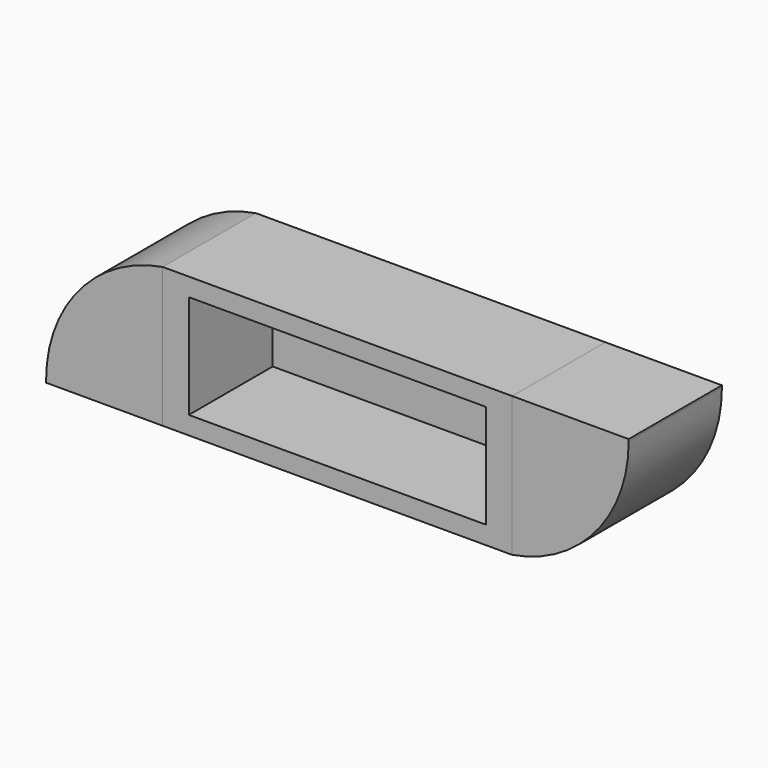
from build123d import *

# Parameters (mm, degrees)
F0_W          = 25.5
F0_H          = 8.9
F1_DEPTH      = 8.9
F2_W          = 30
F2_H          = 12
F2_W_2        = 25.5
F2_H_2        = 8.9
F3_DEPTH      = 10
F4_DEPTH      = 9
F5_DEPTH      = 10
F6_DEPTH      = 10
F9_T1_DEPTH   = 69.160797831
F9_2_T1_DEPTH = 69.160797831


# Not quite as in the source:
# - a fillet or chamfer that OpenCascade refuses, or shapes differently, is made with other operations: its cross-section is extruded or revolved along the edge and cut away or added


with BuildPart() as f1:
    # F0 (on Top) → F1 (new body)
    with BuildSketch(Plane.XY):
        with Locations((12.75, 4.45)):
            Rectangle(F0_W, F0_H)
    extrude(amount=F1_DEPTH)


with BuildPart() as f3:
    # F2 (on face) → F3 (new body)
    with BuildSketch(Plane.XZ):
        with Locations((12.75, 4.45)):
            Rectangle(F2_W, F2_H)
        with Locations((12.75, 4.45)):
            Rectangle(F2_W_2, F2_H_2, mode=Mode.SUBTRACT)
        with Locations((12.75, 4.45)):
            Rectangle(F2_W_2, F2_H_2)
    extrude(amount=-F3_DEPTH)


with BuildPart() as f4_tool:
    # F4 (cut): a face of the model
    f4_faces = [f1.part.faces().sort_by_distance(p)[0] for p in [
        (12.75, 0, 4.45),
    ]]
    extrude(f4_faces, amount=-F4_DEPTH)


with BuildPart() as f1_1:
    add(f1.part)

    # F4: cut by f4_tool
    add(f4_tool.part, mode=Mode.SUBTRACT)


with BuildPart() as f3_1:
    add(f3.part)

    # F4: cut by f4_tool
    add(f4_tool.part, mode=Mode.SUBTRACT)


with BuildPart() as f5:
    # F5 (new): a face of the model
    f5_faces = [f3_1.part.faces().sort_by_distance(p)[0] for p in [
        (-2.25, 5, 4.45),
    ]]
    extrude(f5_faces, amount=F5_DEPTH)

    # F9: fillet of radius 12 on 1 edges, made by hand

    # F9_s2 → F9_t1 (cut)
    with BuildSketch(Plane.XZ.offset(-39.5803989155)):
        with BuildLine():
            ThreePointArc((-2.25, 10.45), (-9.4151513899, 6.3638071262), (-12.25, -1.3821595662))
            Line((-12.25, -1.3821595662), (-12.25, 10.45))
            Line((-12.25, 10.45), (-2.25, 10.45))
        make_face()
    extrude(amount=F9_T1_DEPTH, mode=Mode.SUBTRACT)


with BuildPart() as f6:
    # F6 (new): a face of the model
    f6_faces = [f3_1.part.faces().sort_by_distance(p)[0] for p in [
        (27.75, 5, 4.45),
    ]]
    extrude(f6_faces, amount=F6_DEPTH)

    # F9#2: fillet of radius 12 on 1 edges, made by hand

    # F9_2_s2 → F9_2_t1 (cut)
    with BuildSketch(Plane.XZ.offset(-39.5803989155)):
        with BuildLine():
            ThreePointArc((27.75, -1.55), (34.9151513899, 2.5361928738), (37.75, 10.2821595662))
            Line((37.75, 10.2821595662), (37.75, -1.55))
            Line((37.75, -1.55), (27.75, -1.55))
        make_face()
    extrude(amount=F9_2_T1_DEPTH, mode=Mode.SUBTRACT)


solid = Compound([f3_1.part, f5.part, f6.part])
